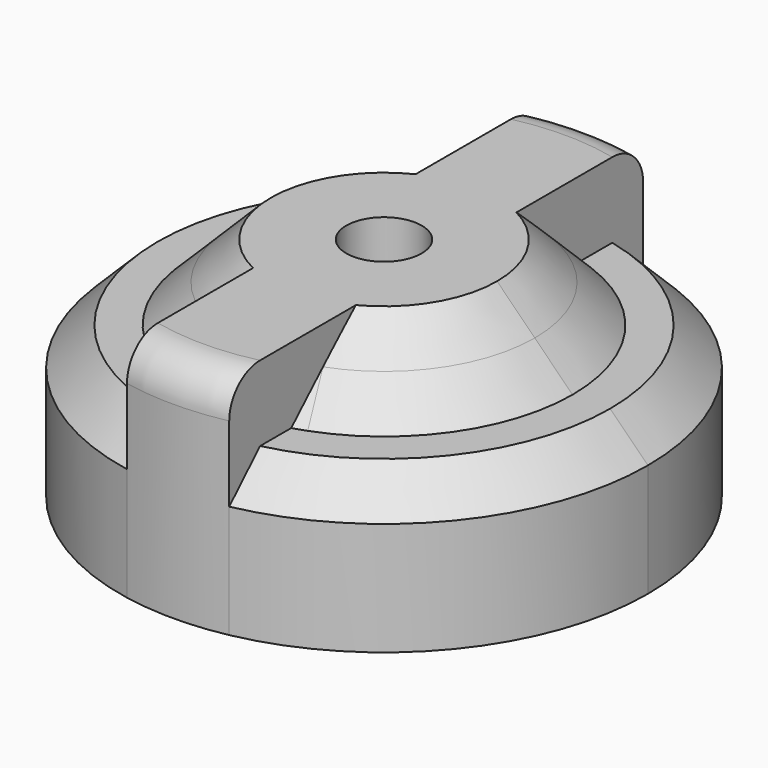
from build123d import *
from build123d import SkipClean  # not in build123d's __all__

# Parameters (mm, degrees)
F0_R     = 3.175
F1_DEPTH = 12.7
F2_DEPTH = 19.05
F3_SIZE  = 3.17499
F4_DEPTH = 19.05
F5_R     = 3.175
F6_START = 6
F6_DEPTH = 15


# Not quite as in the source:
# - a fillet or chamfer is up to 0.001 mm smaller than in the source, because OpenCascade refuses the exact size


with BuildPart() as f1:
    # F0 (on Top) → F1 (new body)
    with BuildSketch(Plane.XY):
        with BuildLine():
            Line((-4.1830006975, 11.9913512652), (-4.1830006975, 21.8278063526))
            ThreePointArc((-4.1830006975, 21.8278063526), (-22.225, 0), (-4.1830006975, -21.8278063526))
            Line((-4.1830006975, -21.8278063526), (-4.1830006975, -11.9913512652))
            ThreePointArc((-4.1830006975, -11.9913512652), (-12.7, 0), (-4.1830006975, 11.9913512652))
        make_face()
        with BuildLine():
            ThreePointArc((4.3927960263, -21.7865547545), (17.1985539608, -14.0769445072), (22.225, 0))
            ThreePointArc((22.225, 0), (17.1985539608, 14.0769445072), (4.3927960263, 21.7865547545))
            Line((4.3927960263, 21.7865547545), (4.3927960263, 11.916095966))
            ThreePointArc((4.3927960263, 11.916095966), (10.4182174467, 7.2629708269), (12.7, 0))
            ThreePointArc((12.7, 0), (10.4182174467, -7.2629708269), (4.3927960263, -11.916095966))
            Line((4.3927960263, -11.916095966), (4.3927960263, -21.7865547545))
        make_face()
        with BuildLine():
            Line((4.3927960263, -11.916095966), (4.3927960263, 11.916095966))
            ThreePointArc((4.3927960263, 11.916095966), (0.1114421824, 12.6995110394), (-4.1830006975, 11.9913512652))
            Line((-4.1830006975, 11.9913512652), (-4.1830006975, -11.9913512652))
            ThreePointArc((-4.1830006975, -11.9913512652), (0.1114421824, -12.6995110394), (4.3927960263, -11.916095966))
        make_face()
        Circle(F0_R, mode=Mode.SUBTRACT)
        with BuildLine():
            Line((-4.1830006975, -11.9913512652), (-4.1830006975, 11.9913512652))
            ThreePointArc((-4.1830006975, 11.9913512652), (-12.7, 0), (-4.1830006975, -11.9913512652))
        make_face()
        with BuildLine():
            ThreePointArc((12.7, 0), (10.4182174467, 7.2629708269), (4.3927960263, 11.916095966))
            Line((4.3927960263, 11.916095966), (4.3927960263, -11.916095966))
            ThreePointArc((4.3927960263, -11.916095966), (10.4182174467, -7.2629708269), (12.7, 0))
        make_face()
        with BuildLine():
            Line((4.3927960263, 11.916095966), (4.3927960263, 21.7865547545))
            ThreePointArc((4.3927960263, 21.7865547545), (0.1069062374, 22.2247428794), (-4.1830006975, 21.8278063526))
            Line((-4.1830006975, 21.8278063526), (-4.1830006975, 11.9913512652))
            ThreePointArc((-4.1830006975, 11.9913512652), (0.1114421824, 12.6995110394), (4.3927960263, 11.916095966))
        make_face()
        with BuildLine():
            ThreePointArc((-4.1830006975, -21.8278063526), (0.1069062374, -22.2247428794), (4.3927960263, -21.7865547545))
            Line((4.3927960263, -21.7865547545), (4.3927960263, -11.916095966))
            ThreePointArc((4.3927960263, -11.916095966), (0.1114421824, -12.6995110394), (-4.1830006975, -11.9913512652))
            Line((-4.1830006975, -11.9913512652), (-4.1830006975, -21.8278063526))
        make_face()
        Circle(F0_R)
    extrude(amount=F1_DEPTH)

    # F0 (on Top) → F2 (join)
    with BuildSketch(Plane.XY):
        with BuildLine():
            ThreePointArc((12.7, 0), (10.4182174467, 7.2629708269), (4.3927960263, 11.916095966))
            Line((4.3927960263, 11.916095966), (4.3927960263, -11.916095966))
            ThreePointArc((4.3927960263, -11.916095966), (10.4182174467, -7.2629708269), (12.7, 0))
        make_face()
        with BuildLine():
            Line((-4.1830006975, -11.9913512652), (-4.1830006975, 11.9913512652))
            ThreePointArc((-4.1830006975, 11.9913512652), (-12.7, 0), (-4.1830006975, -11.9913512652))
        make_face()
        with BuildLine():
            Line((4.3927960263, -11.916095966), (4.3927960263, 11.916095966))
            ThreePointArc((4.3927960263, 11.916095966), (0.1114421824, 12.6995110394), (-4.1830006975, 11.9913512652))
            Line((-4.1830006975, 11.9913512652), (-4.1830006975, -11.9913512652))
            ThreePointArc((-4.1830006975, -11.9913512652), (0.1114421824, -12.6995110394), (4.3927960263, -11.916095966))
        make_face()
        Circle(F0_R, mode=Mode.SUBTRACT)
        Circle(F0_R)
    extrude(amount=F2_DEPTH)

    # F3 (size 3.175 in the source; OpenCascade refuses exactly that, so slightly less here)
    f3_edges = [f1.edges().sort_by_distance(p)[0] for p in [
        (4.183001, -21.827806, 12.7),
        (-4.392796, -11.916096, 12.7),
        (-4.392796, -11.916096, 19.05),
    ]]
    chamfer(f3_edges, length=F3_SIZE)

    # F0 (on Top) → F4 (join)
    with BuildSketch(Plane.XY):
        with BuildLine():
            Line((4.3927960263, 11.916095966), (4.3927960263, 21.7865547545))
            ThreePointArc((4.3927960263, 21.7865547545), (0.1069062374, 22.2247428794), (-4.1830006975, 21.8278063526))
            Line((-4.1830006975, 21.8278063526), (-4.1830006975, 11.9913512652))
            ThreePointArc((-4.1830006975, 11.9913512652), (0.1114421824, 12.6995110394), (4.3927960263, 11.916095966))
        make_face()
        with BuildLine():
            Line((4.3927960263, -11.916095966), (4.3927960263, 11.916095966))
            ThreePointArc((4.3927960263, 11.916095966), (0.1114421824, 12.6995110394), (-4.1830006975, 11.9913512652))
            Line((-4.1830006975, 11.9913512652), (-4.1830006975, -11.9913512652))
            ThreePointArc((-4.1830006975, -11.9913512652), (0.1114421824, -12.6995110394), (4.3927960263, -11.916095966))
        make_face()
        Circle(F0_R, mode=Mode.SUBTRACT)
        with BuildLine():
            ThreePointArc((-4.1830006975, -21.8278063526), (0.1069062374, -22.2247428794), (4.3927960263, -21.7865547545))
            Line((4.3927960263, -21.7865547545), (4.3927960263, -11.916095966))
            ThreePointArc((4.3927960263, -11.916095966), (0.1114421824, -12.6995110394), (-4.1830006975, -11.9913512652))
            Line((-4.1830006975, -11.9913512652), (-4.1830006975, -21.8278063526))
        make_face()
    with SkipClean():  # cleaning this boolean's faces spoils the solid; the shape is the same uncleaned
        extrude(amount=F4_DEPTH)

    # F5
    f5_edges = [f1.edges().sort_by_distance(p)[0] for p in [
        (0.106906, -22.224743, 19.05),
        (0.106906, 22.224743, 19.05),
    ]]
    fillet(f5_edges, radius=F5_R)

    # F0 (on Top) → F6 (cut)
    with BuildSketch(Plane.XY.offset(F6_START)):
        Circle(F0_R)
    extrude(amount=F6_DEPTH, mode=Mode.SUBTRACT)


solid = f1.part
